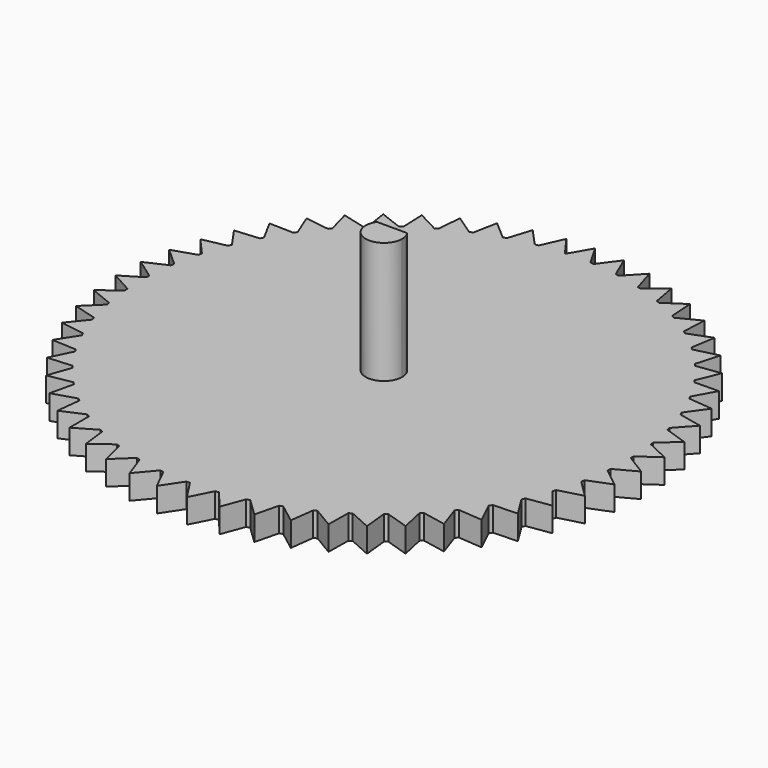
from build123d import *

# Parameters (mm, degrees)
F1_DEPTH = 2
F3_DEPTH = 10


# Not quite as in the source:
# - a feature names something its author has since deleted; it is built from what else it names


with BuildPart() as f1:
    # F0 (on Top) → F1 (new body)
    with BuildSketch(Plane.XY):
        with BuildLine():
            ThreePointArc((19.9343466567, -1.6192045483), (19.9835799237, -0.8102675069), (20, 0))
            ThreePointArc((20, 0), (19.9990981924, 0.1899249575), (19.9963928511, 0.3798327874))
            ThreePointArc((19.9963928511, 0.3798327874), (19.9931464995, 0.5235389662), (19.9888674018, 0.6672181015))
            ThreePointArc((19.9888674018, 0.6672181015), (19.9305047766, 1.665826927), (19.8222847091, 2.6602685791))
            ThreePointArc((19.8222847091, 2.6602685791), (19.802653144, 2.802664528), (19.7819986728, 2.9449157052))
            ThreePointArc((19.7819986728, 2.9449157052), (19.6100099151, 3.9303321907), (19.3889654537, 4.9059166968))
            ThreePointArc((19.3889654537, 4.9059166968), (19.3532053923, 5.0451403392), (19.3164456409, 5.1841033749))
            ThreePointArc((19.3164456409, 5.1841033749), (19.0330798053, 6.1434414725), (18.7021014937, 7.0874113554))
            ThreePointArc((18.7021014937, 7.0874113554), (18.6506805614, 7.2216420983), (18.5982962281, 7.3554998071))
            ThreePointArc((18.5982962281, 7.3554998071), (18.2072588193, 8.2762144901), (17.7706747791, 9.1762256891))
            ThreePointArc((17.7706747791, 9.1762256891), (17.7042653948, 9.3037082302), (17.6369414964, 9.4307101881))
            ThreePointArc((17.6369414964, 9.4307101881), (17.143346014, 10.3007614982), (16.6068653466, 11.1450447895))
            ThreePointArc((16.6068653466, 11.1450447895), (16.5263359293, 11.2641120711), (16.444952844, 11.3825975049))
            ThreePointArc((16.444952844, 11.3825975049), (15.855253914, 12.1906079965), (15.2258920443, 12.9681228963))
            ThreePointArc((15.2258920443, 12.9681228963), (15.1322956573, 13.0772179051), (15.0379176115, 13.1856374101))
            ThreePointArc((15.0379176115, 13.1856374101), (14.3598265809, 13.9210409297), (13.6458135185, 14.6216200682))
            ThreePointArc((13.6458135185, 14.6216200682), (13.5403740986, 14.7193161957), (13.4342352505, 14.8162519968))
            ThreePointArc((13.4342352505, 14.8162519968), (12.676619348, 15.4694318547), (11.887292065, 16.0839139316))
            ThreePointArc((11.887292065, 16.0839139316), (11.7713884175, 16.1689336298), (11.6548767187, 16.2531181215))
            ThreePointArc((11.6548767187, 16.2531181215), (10.8276430999, 16.8155328462), (9.973323434, 17.3358824315))
            ThreePointArc((9.973323434, 17.3358824315), (9.8484712021, 17.4071139188), (9.7231102472, 17.4774462414))
            ThreePointArc((9.7231102472, 17.4774462414), (8.8370764416, 17.9417412746), (7.9289361197, 18.3611538856))
            ThreePointArc((7.9289361197, 18.3611538856), (7.7967679652, 18.4176656854), (7.6641970684, 18.4732261204))
            ThreePointArc((7.6641970684, 18.4732261204), (6.7309495209, 18.8333299909), (5.7808640693, 19.1463210725))
            ThreePointArc((5.7808640693, 19.1463210725), (5.6431083224, 19.187374194), (5.5050610806, 19.2274361915))
            ThreePointArc((5.5050610806, 19.2274361915), (4.5368036385, 19.4786399101), (3.5571970896, 19.6811165554))
            ThreePointArc((3.5571970896, 19.6811165554), (3.4156551481, 19.7061741571), (3.2739367709, 19.7302138361))
            ThreePointArc((3.2739367709, 19.7302138361), (2.2833310972, 19.8692324739), (1.2870135235, 19.9585469459))
            ThreePointArc((1.2870135235, 19.9585469459), (1.1435362965, 19.9672813557), (1, 19.9749843554))
            ThreePointArc((1, 19.9749843554), (0, 20), (-1, 19.9749843554))
            ThreePointArc((-1, 19.9749843554), (-1.0467191249, 19.9725906951), (-1.0934325231, 19.9700877644))
            ThreePointArc((-1.0934325231, 19.9700877644), (-2.0905692654, 19.8904379074), (-3.0824763138, 19.7610308379))
            ThreePointArc((-3.0824763138, 19.7610308379), (-3.2244211207, 19.7383664075), (-3.3661993701, 19.7146823916))
            ThreePointArc((-3.3661993701, 19.7146823916), (-4.3477231073, 19.5217136487), (-5.318370735, 19.2799100808))
            ThreePointArc((-5.318370735, 19.2799100808), (-5.4567999333, 19.2411884895), (-5.5949472607, 19.2014729943))
            ThreePointArc((-5.5949472607, 19.2014729943), (-6.5480228498, 18.8977087701), (-7.4847181377, 18.5466707093))
            ThreePointArc((-7.4847181377, 18.5466707093), (-7.6178215232, 18.4923983096), (-7.75053141, 18.4371706848))
            ThreePointArc((-7.75053141, 18.4371706848), (-8.6626957173, 18.0265832289), (-9.5531897329, 17.5709011131))
            ThreePointArc((-9.5531897329, 17.5709011131), (-9.6792267455, 17.5017876118), (-9.8047637775, 17.4317700555))
            ThreePointArc((-9.8047637775, 17.4317700555), (-10.664088656, 16.9197285184), (-11.4967366294, 16.3653611899))
            ThreePointArc((-11.4967366294, 16.3653611899), (-11.6140591142, 16.2823103671), (-11.7307816747, 16.1984184815))
            ThreePointArc((-11.7307816747, 16.1984184815), (-12.5260299455, 15.5916187038), (-13.2899435451, 14.9458154869))
            ThreePointArc((-13.2899435451, 14.9458154869), (-13.397017305, 14.8499133778), (-13.5033990419, 14.7532441963))
            ThreePointArc((-13.5033990419, 14.7532441963), (-14.2241714402, 14.0596211485), (-14.9093611568, 13.3308270522))
            ThreePointArc((-14.9093611568, 13.3308270522), (-15.0047860148, 13.2233277449), (-15.0994358005, 13.1151453865))
            ThreePointArc((-15.0994358005, 13.1151453865), (-15.7363069638, 12.3437694057), (-16.333812741, 11.5415146901))
            ThreePointArc((-16.333812741, 11.5415146901), (-16.4163408499, 11.4238239264), (-16.4980209724, 11.305543065))
            ThreePointArc((-16.4980209724, 11.305543065), (-17.0426626942, 10.466501244), (-17.5446710968, 9.6012767955))
            ThreePointArc((-17.5446710968, 9.6012767955), (-17.6132232568, 9.4749335885), (-17.6808656055, 9.3481009536))
            ThreePointArc((-17.6808656055, 9.3481009536), (-18.1261557407, 8.4523652348), (-18.526102129, 7.5354853796))
            ThreePointArc((-18.526102129, 7.5354853796), (-18.5797819005, 7.402141888), (-18.6325019331, 7.2684160387))
            ThreePointArc((-18.6325019331, 7.2684160387), (-18.9726175328, 6.3276997365), (-19.2652719068, 5.3711542855))
            ThreePointArc((-19.2652719068, 5.3711542855), (-19.3033773327, 5.2325542093), (-19.3404856424, 5.0936838454))
            ThreePointArc((-19.3404856424, 5.0936838454), (-19.5709790989, 4.1202884741), (-19.7525144898, 3.1365859355))
            ThreePointArc((-19.7525144898, 3.1365859355), (-19.7745472749, 2.9945417136), (-19.7955586055, 2.8523428086))
            ThreePointArc((-19.7955586055, 2.8523428086), (-19.913415813, 1.8589972186), (-19.9814583273, 0.8610012273))
            ThreePointArc((-19.9814583273, 0.8610012273), (-19.9871303543, 0.7173703367), (-19.9917699458, 0.5737023904))
            ThreePointArc((-19.9917699458, 0.5737023904), (-19.9954497148, -0.4266036836), (-19.9491095775, -1.4258425811))
            ThreePointArc((-19.9491095775, -1.4258425811), (-19.9383466747, -1.5691819146), (-19.9265538563, -1.7124401919))
            ThreePointArc((-19.9265538563, -1.7124401919), (-19.8160080673, -2.706625995), (-19.6558912568, -3.6940409987))
            ThreePointArc((-19.6558912568, -3.6940409987), (-19.628834168, -3.8352143621), (-19.6007631516, -3.9761896176))
            ThreePointArc((-19.6007631516, -3.9761896176), (-19.3774373845, -4.9512544278), (-19.1056377088, -5.913933356))
            ThreePointArc((-19.1056377088, -5.913933356), (-19.0626402529, -6.0510946603), (-19.0186581161, -6.1879433952))
            ThreePointArc((-19.0186581161, -6.1879433952), (-18.6854727468, -7.1311365314), (-18.305544463, -8.0564906699))
            ThreePointArc((-18.305544463, -8.0564906699), (-18.2471689071, -8.1878462905), (-18.1878507934, -8.3187789679))
            ThreePointArc((-18.1878507934, -8.3187789679), (-17.7491628045, -9.2177665267), (-17.2660741408, -10.0936952483))
            ThreePointArc((-17.2660741408, -10.0936952483), (-17.1930838475, -10.2175274804), (-17.1192054453, -10.3408319259))
            ThreePointArc((-17.1192054453, -10.3408319259), (-16.5807514511, -11.1838580694), (-16.0008196384, -11.9989070711))
            ThreePointArc((-16.0008196384, -11.9989070711), (-15.9141690838, -12.1135965911), (-15.8266964827, -12.2276603831))
            ThreePointArc((-15.8266964827, -12.2276603831), (-15.1955177129, -13.0037010669), (-14.526326376, -13.7472121544))
            ThreePointArc((-14.526326376, -13.7472121544), (-14.427148668, -13.8512591959), (-14.3272257255, -13.9545907504))
            ThreePointArc((-14.3272257255, -13.9545907504), (-13.6115759486, -14.6534978826), (-12.8618759372, -15.3157483453))
            ThreePointArc((-12.8618759372, -15.3157483453), (-12.7514679981, -15.4077923108), (-12.6404013818, -15.4990403866))
            ThreePointArc((-12.6404013818, -15.4990403866), (-11.8496389731, -16.1116745315), (-11.0292339287, -16.6840042839))
            ThreePointArc((-11.0292339287, -16.6840042839), (-10.9090395358, -16.7628415374), (-10.7882816364, -16.840812906))
            ThreePointArc((-10.7882816364, -16.840812906), (-9.9327472001, -17.3591627983), (-9.0523653565, -17.834087626))
            ThreePointArc((-9.0523653565, -17.834087626), (-8.9239562622, -17.898687232), (-8.7950862008, -17.9623622812))
            ThreePointArc((-8.7950862008, -17.9623622812), (-7.8859673492, -18.3796495877), (-6.957121242, -18.7509590161))
            ThreePointArc((-6.957121242, -18.7509590161), (-6.8221766202, -18.8004762217), (-6.6868795988, -18.8490222885))
            ThreePointArc((-6.6868795988, -18.8490222885), (-5.7360646542, -19.1597902463), (-4.7709005742, -19.4226287539))
            ThreePointArc((-4.7709005742, -19.4226287539), (-4.6311850623, -19.4564160348), (-4.4912303265, -19.4891982943))
            ThreePointArc((-4.4912303265, -19.4891982943), (-3.5111528608, -19.6893830677), (-2.5222920198, -19.8403135804))
            ThreePointArc((-2.5222920198, -19.8403135804), (-2.379632643, -19.8579291087), (-2.2368503464, -19.8745188754))
            ThreePointArc((-2.2368503464, -19.8745188754), (-1.2403265899, -19.9615026977), (-0.2407000766, -19.9985515344))
            ThreePointArc((-0.2407000766, -19.9985515344), (-0.0969623564, -19.9997649562), (0.0467803724, -19.9999452898))
            ThreePointArc((0.0467803724, -19.9999452898), (1.0467191249, -19.9725906951), (2.0440394419, -19.8952733774))
            ThreePointArc((2.0440394419, -19.8952733774), (2.186975883, -19.880068825), (2.3297993559, -19.8638373675))
            ThreePointArc((2.3297993559, -19.8638373675), (3.3200771526, -19.7225020649), (4.3020495623, -19.5318296522))
            ThreePointArc((4.3020495623, -19.5318296522), (4.4423155798, -19.5004059519), (4.5823521295, -19.4679749579))
            ThreePointArc((4.5823521295, -19.4679749579), (5.5500193528, -19.2145071543), (6.5038028449, -18.9129730226))
            ThreePointArc((6.5038028449, -18.9129730226), (6.6395642148, -18.8657410943), (6.7749826179, -18.8175346559))
            ThreePointArc((6.7749826179, -18.8175346559), (7.7073853228, -18.4552488871), (8.6205075066, -18.0467961236))
            ThreePointArc((8.6205075066, -18.0467961236), (8.749988911, -17.9843736076), (8.8790183347, -17.9210221085))
            ThreePointArc((8.8790183347, -17.9210221085), (9.7639637218, -17.4546558958), (10.6244839243, -16.9446257363))
            ThreePointArc((10.6244839243, -16.9446257363), (10.7459921669, -16.8678289163), (10.8669453253, -16.7901607883))
            ThreePointArc((10.8669453253, -16.7901607883), (11.6928611826, -16.2258126873), (12.489526594, -15.6208746701))
            ThreePointArc((12.489526594, -15.6208746701), (12.6014727417, -15.5307077991), (12.7127679602, -15.4397386892))
            ThreePointArc((12.7127679602, -15.4397386892), (13.4688539904, -14.7847885405), (14.1912468142, -14.0928532902))
            ThreePointArc((14.1912468142, -14.0928532902), (14.2921669748, -13.9904954581), (14.3923488734, -13.8874149469))
            ThreePointArc((14.3923488734, -13.8874149469), (15.0687179266, -13.1504273714), (15.7073916105, -12.3805431542))
            ThreePointArc((15.7073916105, -12.3805431542), (15.7959660761, -12.2673328691), (15.8837246009, -12.1534889148))
            ThreePointArc((15.8837246009, -12.1534889148), (16.4715319662, -11.3441013168), (17.0181347326, -10.5063357182))
            ThreePointArc((17.0181347326, -10.5063357182), (17.0932052368, -10.383753403), (17.1673927912, -10.2606347148))
            ThreePointArc((17.1673927912, -10.2606347148), (17.6589518572, -9.3894312557), (18.1063359168, -8.4947395291))
            ThreePointArc((18.1063359168, -8.4947395291), (18.1669207812, -8.3643881624), (18.226567233, -8.233604733))
            ThreePointArc((18.226567233, -8.233604733), (18.6154500033, -7.3119779249), (18.9577650255, -6.3720597327))
            ThreePointArc((18.9577650255, -6.3720597327), (19.0030719968, -6.235643887), (19.0473973641, -6.098905939))
            ThreePointArc((19.0473973641, -6.098905939), (19.328518515, -5.1389076677), (19.5612881309, -4.1660540875))
            ThreePointArc((19.5612881309, -4.1660540875), (19.590724741, -4.0253576391), (19.619149392, -3.8844532608))
            ThreePointArc((19.619149392, -3.8844532608), (19.7888327716, -2.8986371861), (19.9090131106, -1.9055699837))
            ThreePointArc((19.9090131106, -1.9055699837), (19.9221944242, -1.7624327853), (19.9343466567, -1.6192045483))
        make_face()
        with BuildLine():
            Line((-1.3461906451, -21.6652520483), (-0.2407000766, -19.9985515344))
            ThreePointArc((-0.2407000766, -19.9985515344), (-1.2403265899, -19.9615026977), (-2.2368503464, -19.8745188754))
            Line((-2.2368503464, -19.8745188754), (-1.3461906451, -21.6652520483))
        make_face()
        with BuildLine():
            ThreePointArc((15.2258920443, 12.9681228963), (15.855253914, 12.1906079965), (16.444952844, 11.3825975049))
            Line((16.444952844, 11.3825975049), (17.2085277115, 13.2310978219))
            Line((17.2085277115, 13.2310978219), (15.2258920443, 12.9681228963))
        make_face()
        with BuildLine():
            ThreePointArc((13.6458135185, 14.6216200682), (14.3598265809, 13.9210409297), (15.0379176115, 13.1856374101))
            Line((15.0379176115, 13.1856374101), (15.5854630263, 15.1092262484))
            Line((15.5854630263, 15.1092262484), (13.6458135185, 14.6216200682))
        make_face()
        with BuildLine():
            Line((3.6034515748, -21.4058522913), (4.3020495623, -19.5318296522))
            ThreePointArc((4.3020495623, -19.5318296522), (3.3200771526, -19.7225020649), (2.3297993559, -19.8638373675))
            Line((2.3297993559, -19.8638373675), (3.6034515748, -21.4058522913))
        make_face()
        with BuildLine():
            ThreePointArc((-19.9814583273, 0.8610012273), (-19.913415813, 1.8589972186), (-19.7955586055, 2.8523428086))
            Line((-19.7955586055, 2.8523428086), (-21.6130608634, 2.0176658996))
            Line((-21.6130608634, 2.0176658996), (-19.9814583273, 0.8610012273))
        make_face()
        with BuildLine():
            ThreePointArc((11.887292065, 16.0839139316), (12.676619348, 15.4694318547), (13.4342352505, 14.8162519968))
            Line((13.4342352505, 14.8162519968), (13.7585910967, 16.7897750611))
            Line((13.7585910967, 16.7897750611), (11.887292065, 16.0839139316))
        make_face()
        with BuildLine():
            Line((-21.702096503, -0.4630150581), (-19.9491095775, -1.4258425811))
            ThreePointArc((-19.9491095775, -1.4258425811), (-19.9954497148, -0.4266036836), (-19.9917699458, 0.5737023904))
            Line((-19.9917699458, 0.5737023904), (-21.702096503, -0.4630150581))
        make_face()
        with BuildLine():
            ThreePointArc((17.7706747791, 9.1762256891), (18.2072588193, 8.2762144901), (18.5982962281, 7.3554998071))
            Line((18.5982962281, 7.3554998071), (19.7612803707, 8.9826039477))
            Line((19.7612803707, 8.9826039477), (17.7706747791, 9.1762256891))
        make_face()
        with BuildLine():
            Line((16.3548594947, -14.272839468), (15.7073916105, -12.3805431542))
            ThreePointArc((15.7073916105, -12.3805431542), (15.0687179266, -13.1504273714), (14.3923488734, -13.8874149469))
            Line((14.3923488734, -13.8874149469), (16.3548594947, -14.272839468))
        make_face()
        with BuildLine():
            ThreePointArc((18.7021014937, 7.0874113554), (19.0330798053, 6.1434414725), (19.3164456409, 5.1841033749))
            Line((19.3164456409, 5.1841033749), (20.6575866297, 6.6677950033))
            Line((20.6575866297, 6.6677950033), (18.7021014937, 7.0874113554))
        make_face()
        with BuildLine():
            Line((1.1360584425, -21.6772864257), (2.0440394419, -19.8952733774))
            ThreePointArc((2.0440394419, -19.8952733774), (1.0467191249, -19.9725906951), (0.0467803724, -19.9999452898))
            Line((0.0467803724, -19.9999452898), (1.1360584425, -21.6772864257))
        make_face()
        with BuildLine():
            Line((12.6908674423, -17.6107143276), (12.489526594, -15.6208746701))
            ThreePointArc((12.489526594, -15.6208746701), (11.6928611826, -16.2258126873), (10.8669453253, -16.7901607883))
            Line((10.8669453253, -16.7901607883), (12.6908674423, -17.6107143276))
        make_face()
        with BuildLine():
            Line((14.6184443587, -16.0466962363), (14.1912468142, -14.0928532902))
            ThreePointArc((14.1912468142, -14.0928532902), (13.4688539904, -14.7847885405), (12.7127679602, -15.4397386892))
            Line((12.7127679602, -15.4397386892), (14.6184443587, -16.0466962363))
        make_face()
        with BuildLine():
            Line((-21.5073391954, -2.9376412823), (-19.6558912568, -3.6940409987))
            ThreePointArc((-19.6558912568, -3.6940409987), (-19.8160080673, -2.706625995), (-19.9265538563, -1.7124401919))
            Line((-19.9265538563, -1.7124401919), (-21.5073391954, -2.9376412823))
        make_face()
        with BuildLine():
            ThreePointArc((7.9289361197, 18.3611538856), (8.8370764416, 17.9417412746), (9.7231102472, 17.4774462414))
            Line((9.7231102472, 17.4774462414), (9.5913364528, 19.4731004367))
            Line((9.5913364528, 19.4731004367), (7.9289361197, 18.3611538856))
        make_face()
        with BuildLine():
            Line((8.3652242109, -20.0304368267), (8.6205075066, -18.0467961236))
            ThreePointArc((8.6205075066, -18.0467961236), (7.7073853228, -18.4552488871), (6.7749826179, -18.8175346559))
            Line((6.7749826179, -18.8175346559), (8.3652242109, -20.0304368267))
        make_face()
        with BuildLine():
            ThreePointArc((9.973323434, 17.3358824315), (10.8276430999, 16.8155328462), (11.6548767187, 16.2531181215))
            Line((11.6548767187, 16.2531181215), (11.7518014751, 18.2507681388))
            Line((11.7518014751, 18.2507681388), (9.973323434, 17.3358824315))
        make_face()
        with BuildLine():
            ThreePointArc((3.5571970896, 19.6811165554), (4.5368036385, 19.4786399101), (5.5050610806, 19.2274361915))
            Line((5.5050610806, 19.2274361915), (4.9240278054, 21.1411760728))
            Line((4.9240278054, 21.1411760728), (3.5571970896, 19.6811165554))
        make_face()
        with BuildLine():
            ThreePointArc((16.6068653466, 11.1450447895), (17.143346014, 10.3007614982), (17.6369414964, 9.4307101881))
            Line((17.6369414964, 9.4307101881), (18.6065607369, 11.1799496024))
            Line((18.6065607369, 11.1799496024), (16.6068653466, 11.1450447895))
        make_face()
        with BuildLine():
            Line((6.0237232623, -20.8544991219), (6.5038028449, -18.9129730226))
            ThreePointArc((6.5038028449, -18.9129730226), (5.5500193528, -19.2145071543), (4.5823521295, -19.4679749579))
            Line((4.5823521295, -19.4679749579), (6.0237232623, -20.8544991219))
        make_face()
        with BuildLine():
            Line((17.877406179, -12.3123403088), (17.0181347326, -10.5063357182))
            ThreePointArc((17.0181347326, -10.5063357182), (16.4715319662, -11.3441013168), (15.8837246009, -12.1534889148))
            Line((15.8837246009, -12.1534889148), (17.877406179, -12.3123403088))
        make_face()
        with BuildLine():
            Line((19.1661744453, -10.1908357214), (18.1063359168, -8.4947395291))
            ThreePointArc((18.1063359168, -8.4947395291), (17.6589518572, -9.3894312557), (17.1673927912, -10.2606347148))
            Line((17.1673927912, -10.2606347148), (19.1661744453, -10.1908357214))
        make_face()
        with BuildLine():
            Line((-17.9959477389, -12.1384200185), (-16.0008196384, -11.9989070711))
            ThreePointArc((-16.0008196384, -11.9989070711), (-16.5807514511, -11.1838580694), (-17.1192054453, -10.3408319259))
            Line((-17.1192054453, -10.3408319259), (-17.9959477389, -12.1384200185))
        make_face()
        with BuildLine():
            ThreePointArc((-1, 19.9749843554), (0, 20), (1, 19.9749843554))
            Line((1, 19.9749843554), (0, 21.707035163))
            Line((0, 21.707035163), (-1, 19.9749843554))
        make_face()
        with BuildLine():
            Line((-10.7805246369, -18.8407978632), (-9.0523653565, -17.834087626))
            ThreePointArc((-9.0523653565, -17.834087626), (-9.9327472001, -17.3591627983), (-10.7882816364, -16.840812906))
            Line((-10.7882816364, -16.840812906), (-10.7805246369, -18.8407978632))
        make_face()
        with BuildLine():
            Line((-12.8610264929, -17.4868342795), (-11.0292339287, -16.6840042839))
            ThreePointArc((-11.0292339287, -16.6840042839), (-11.8496389731, -16.1116745315), (-12.6404013818, -15.4990403866))
            Line((-12.6404013818, -15.4990403866), (-12.8610264929, -17.4868342795))
        make_face()
        with BuildLine():
            Line((21.4778444404, -3.1460409662), (19.9090131106, -1.9055699837))
            ThreePointArc((19.9090131106, -1.9055699837), (19.7888327716, -2.8986371861), (19.619149392, -3.8844532608))
            Line((19.619149392, -3.8844532608), (21.4778444404, -3.1460409662))
        make_face()
        with BuildLine():
            ThreePointArc((1.2870135235, 19.9585469459), (2.2833310972, 19.8692324739), (3.2739367709, 19.7302138361))
            Line((3.2739367709, 19.7302138361), (2.4782174208, 21.5651063986))
            Line((2.4782174208, 21.5651063986), (1.2870135235, 19.9585469459))
        make_face()
        with BuildLine():
            Line((10.5973351919, -18.9444414644), (10.6244839243, -16.9446257363))
            ThreePointArc((10.6244839243, -16.9446257363), (9.7639637218, -17.4546558958), (8.8790183347, -17.9210221085))
            Line((8.8790183347, -17.9210221085), (10.5973351919, -18.9444414644))
        make_face()
        with BuildLine():
            Line((-3.8108359306, -21.3699065295), (-2.5222920198, -19.8403135804))
            ThreePointArc((-2.5222920198, -19.8403135804), (-3.5111528608, -19.6893830677), (-4.4912303265, -19.4891982943))
            Line((-4.4912303265, -19.4891982943), (-3.8108359306, -21.3699065295))
        make_face()
        with BuildLine():
            Line((-16.4924818656, -14.1135898155), (-14.526326376, -13.7472121544))
            ThreePointArc((-14.526326376, -13.7472121544), (-15.1955177129, -13.0037010669), (-15.8266964827, -12.2276603831))
            Line((-15.8266964827, -12.2276603831), (-16.4924818656, -14.1135898155))
        make_face()
        with BuildLine():
            Line((-19.2640850555, -10.0045191059), (-17.2660741408, -10.0936952483))
            ThreePointArc((-17.2660741408, -10.0936952483), (-17.7491628045, -9.2177665267), (-18.1878507934, -8.3187789679))
            Line((-18.1878507934, -8.3187789679), (-19.2640850555, -10.0045191059))
        make_face()
        with BuildLine():
            ThreePointArc((19.8222847091, 2.6602685791), (19.9305047766, 1.665826927), (19.9888674018, 0.6672181015))
            Line((19.9888674018, 0.6672181015), (21.6316084001, 1.808008184))
            Line((21.6316084001, 1.808008184), (19.8222847091, 2.6602685791))
        make_face()
        with BuildLine():
            ThreePointArc((19.9963928511, 0.3798327874), (19.9990981924, 0.1899249575), (20, 0))
            ThreePointArc((20, 0), (19.9835799237, -0.8102675069), (19.9343466567, -1.6192045483))
            Line((19.9343466567, -1.6192045483), (21.6965868698, -0.6734194609))
            Line((21.6965868698, -0.6734194609), (19.9963928511, 0.3798327874))
        make_face()
        with BuildLine():
            Line((20.9782415527, -5.5775224721), (19.5612881309, -4.1660540875))
            ThreePointArc((19.5612881309, -4.1660540875), (19.328518515, -5.1389076677), (19.0473973641, -6.098905939))
            Line((19.0473973641, -6.098905939), (20.9782415527, -5.5775224721))
        make_face()
        with BuildLine():
            Line((-14.7733478871, -15.9041996899), (-12.8618759372, -15.3157483453))
            ThreePointArc((-12.8618759372, -15.3157483453), (-13.6115759486, -14.6534978826), (-14.3272257255, -13.9545907504))
            Line((-14.3272257255, -13.9545907504), (-14.7733478871, -15.9041996899))
        make_face()
        with BuildLine():
            Line((-8.5590485272, -19.9483849942), (-6.957121242, -18.7509590161))
            ThreePointArc((-6.957121242, -18.7509590161), (-7.8859673492, -18.3796495877), (-8.7950862008, -17.9623622812))
            Line((-8.7950862008, -17.9623622812), (-8.5590485272, -19.9483849942))
        make_face()
        with BuildLine():
            Line((20.2043113899, -7.9360680964), (18.9577650255, -6.3720597327))
            ThreePointArc((18.9577650255, -6.3720597327), (18.6154500033, -7.3119779249), (18.226567233, -8.233604733))
            Line((18.226567233, -8.233604733), (20.2043113899, -7.9360680964))
        make_face()
        with BuildLine():
            Line((-6.2256478573, -20.7951120296), (-4.7709005742, -19.4226287539))
            ThreePointArc((-4.7709005742, -19.4226287539), (-5.7360646542, -19.1597902463), (-6.6868795988, -18.8490222885))
            Line((-6.6868795988, -18.8490222885), (-6.2256478573, -20.7951120296))
        make_face()
        with BuildLine():
            ThreePointArc((5.7808640693, 19.1463210725), (6.7309495209, 18.8333299909), (7.6641970684, 18.4732261204))
            Line((7.6641970684, 18.4732261204), (7.3054478966, 20.4407878175))
            Line((7.3054478966, 20.4407878175), (5.7808640693, 19.1463210725))
        make_face()
        with BuildLine():
            ThreePointArc((-19.7525144898, 3.1365859355), (-19.5709790989, 4.1202884741), (-19.3404856424, 5.0936838454))
            Line((-19.3404856424, 5.0936838454), (-21.2413965737, 4.4719623394))
            Line((-21.2413965737, 4.4719623394), (-19.7525144898, 3.1365859355))
        make_face()
        with BuildLine():
            ThreePointArc((19.3889654537, 4.9059166968), (19.6100099151, 3.9303321907), (19.7819986728, 2.9449157052))
            Line((19.7819986728, 2.9449157052), (21.2837587387, 4.2657929532))
            Line((21.2837587387, 4.2657929532), (19.3889654537, 4.9059166968))
        make_face()
        with BuildLine():
            Line((-20.2803106976, -7.7397915719), (-18.305544463, -8.0564906699))
            ThreePointArc((-18.305544463, -8.0564906699), (-18.6854727468, -7.1311365314), (-19.0186581161, -6.1879433952))
            Line((-19.0186581161, -6.1879433952), (-20.2803106976, -7.7397915719))
        make_face()
        with BuildLine():
            ThreePointArc((-13.2899435451, 14.9458154869), (-12.5260299455, 15.5916187038), (-11.7307816747, 16.1984184815))
            Line((-11.7307816747, 16.1984184815), (-13.595148624, 16.9223907725))
            Line((-13.595148624, 16.9223907725), (-13.2899435451, 14.9458154869))
        make_face()
        with BuildLine():
            ThreePointArc((-18.526102129, 7.5354853796), (-18.1261557407, 8.4523652348), (-17.6808656055, 9.3481009536))
            Line((-17.6808656055, 9.3481009536), (-19.6732550017, 9.1737894681))
            Line((-19.6732550017, 9.1737894681), (-18.526102129, 7.5354853796))
        make_face()
        with BuildLine():
            ThreePointArc((-16.333812741, 11.5415146901), (-15.7363069638, 12.3437694057), (-15.0994358005, 13.1151453865))
            Line((-15.0994358005, 13.1151453865), (-17.07942843, 13.3973318266))
            Line((-17.07942843, 13.3973318266), (-16.333812741, 11.5415146901))
        make_face()
        with BuildLine():
            ThreePointArc((-14.9093611568, 13.3308270522), (-14.2241714402, 14.0596211485), (-13.5033990419, 14.7532441963))
            Line((-13.5033990419, 14.7532441963), (-15.4382294809, 15.2596345325))
            Line((-15.4382294809, 15.2596345325), (-14.9093611568, 13.3308270522))
        make_face()
        with BuildLine():
            Line((-21.0313357337, -5.3738526983), (-19.1056377088, -5.913933356))
            ThreePointArc((-19.1056377088, -5.913933356), (-19.3774373845, -4.9512544278), (-19.6007631516, -3.9761896176))
            Line((-19.6007631516, -3.9761896176), (-21.0313357337, -5.3738526983))
        make_face()
        with BuildLine():
            ThreePointArc((-19.2652719068, 5.3711542855), (-18.9726175328, 6.3276997365), (-18.6325019331, 7.2684160387))
            Line((-18.6325019331, 7.2684160387), (-20.5919637959, 6.867780034))
            Line((-20.5919637959, 6.867780034), (-19.2652719068, 5.3711542855))
        make_face()
        with BuildLine():
            ThreePointArc((-17.5446710968, 9.6012767955), (-17.0426626942, 10.466501244), (-16.4980209724, 11.305543065))
            Line((-16.4980209724, 11.305543065), (-18.4972839188, 11.3598355268))
            Line((-18.4972839188, 11.3598355268), (-17.5446710968, 9.6012767955))
        make_face()
        with BuildLine():
            ThreePointArc((-11.4967366294, 16.3653611899), (-10.664088656, 16.9197285184), (-9.8047637775, 17.4317700555))
            Line((-9.8047637775, 17.4317700555), (-11.5742873719, 18.3638570949))
            Line((-11.5742873719, 18.3638570949), (-11.4967366294, 16.3653611899))
        make_face()
        with BuildLine():
            ThreePointArc((-9.5531897329, 17.5709011131), (-8.6626957173, 18.0265832289), (-7.75053141, 18.4371706848))
            Line((-7.75053141, 18.4371706848), (-9.4020720271, 19.5651838009))
            Line((-9.4020720271, 19.5651838009), (-9.5531897329, 17.5709011131))
        make_face()
        with BuildLine():
            ThreePointArc((-7.4847181377, 18.5466707093), (-6.5480228498, 18.8977087701), (-5.5949472607, 19.2014729943))
            Line((-5.5949472607, 19.2014729943), (-7.1069081124, 20.5106614386))
            Line((-7.1069081124, 20.5106614386), (-7.4847181377, 18.5466707093))
        make_face()
        with BuildLine():
            ThreePointArc((-5.318370735, 19.2799100808), (-4.3477231073, 19.5217136487), (-3.3661993701, 19.7146823916))
            Line((-3.3661993701, 19.7146823916), (-4.7188089185, 21.1879262307))
            Line((-4.7188089185, 21.1879262307), (-5.318370735, 19.2799100808))
        make_face()
        with BuildLine():
            ThreePointArc((-3.0824763138, 19.7610308379), (-2.0905692654, 19.8904379074), (-1.0934325231, 19.9700877644))
            Line((-1.0934325231, 19.9700877644), (-2.2690030277, 21.5881217531))
            Line((-2.2690030277, 21.5881217531), (-3.0824763138, 19.7610308379))
        make_face()
    extrude(amount=F1_DEPTH)

    # F2 (on face) → F3 (join)
    with BuildSketch(Plane.XY.offset(2)):
        with BuildLine():
            ThreePointArc((-1.25, 0.8291561976), (-0.4330127019, -1.4361406616), (1.5, 0))
            ThreePointArc((1.5, 0), (1.4361406616, 0.4330127019), (1.25, 0.8291561976))
            Line((1.25, 0.8291561976), (-1.25, 0.8291561976))
        make_face()
    extrude(amount=F3_DEPTH)


solid = f1.part
